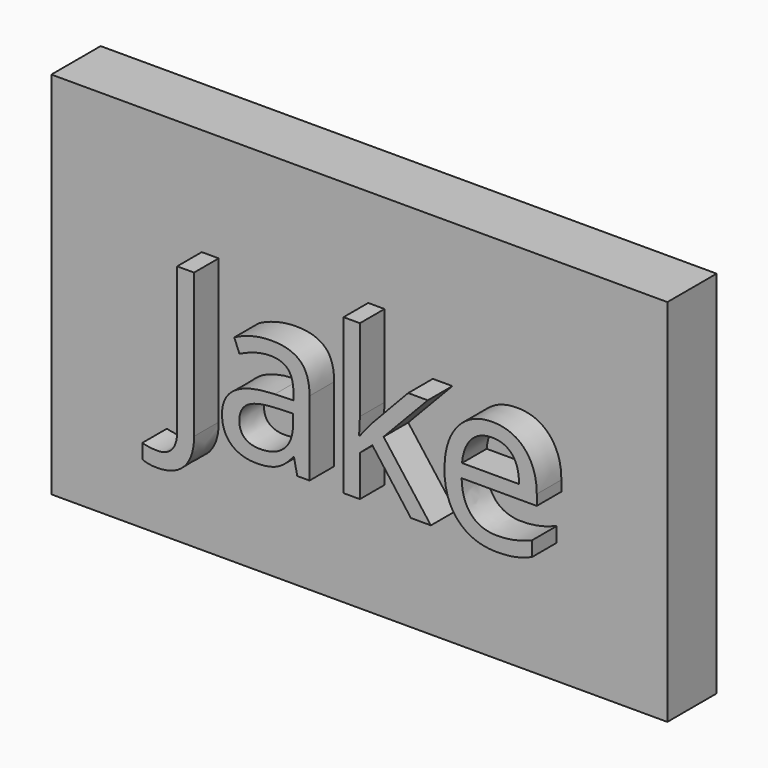
from build123d import *

# Parameters (mm, degrees)
F0_W         = 63.5
F0_H         = 38.1
F1_DEPTH     = 6.35
F2_TEXT_SIZE = 21.0167089891
F3_DEPTH     = 3.175


# Not quite as in the source:
# - Text() gives the source's letters only with a copy of the font that has no kerning and outlines rounded to 1/6400 em; it was checked with that copy


with BuildPart() as f1:
    # F0 (on Front) → F1 (new body)
    with BuildSketch(Plane.XZ):
        with Locations((31.75, 19.05)):
            Rectangle(F0_W, F0_H)
    extrude(amount=F1_DEPTH)

    # F2 (on face) → F3 (join)
    with BuildSketch(Plane.XZ.offset(6.35)):
        with Locations((13.555534184, 12.0244137943)):
            Text('Jake', F2_TEXT_SIZE, font='Open Sans', text_align=(TextAlign.LEFT, TextAlign.BOTTOM))
    extrude(amount=F3_DEPTH)


solid = f1.part
